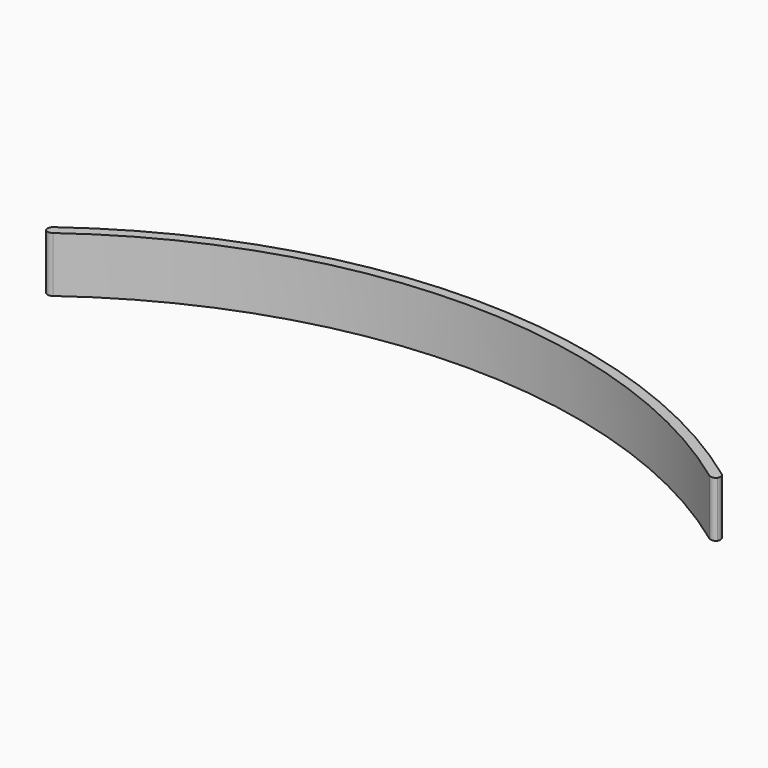
from build123d import *

# Parameters (mm, degrees)
F1_DEPTH    = 25
F2_T1_DEPTH = 37.6241632485
F2_T3_DEPTH = 37.4381172953


# Not quite as in the source:
# - a fillet or chamfer that OpenCascade refuses, or shapes differently, is made with other operations: its cross-section is extruded or revolved along the edge and cut away or added


with BuildPart() as f1:
    # F0 (on Top) → F1 (new body)
    with BuildSketch(Plane.XY):
        with BuildLine():
            ThreePointArc((-150, 0), (0, 50), (150, 0))
            Line((150, 0), (152.7, 3.6))
            ThreePointArc((152.7, 3.6), (0, 54.5), (-152.7, 3.6))
            Line((-152.7, 3.6), (-150, 0))
        make_face()
    extrude(amount=F1_DEPTH)

    # F2: fillet of radius 2.5 on 4 edges, made by hand

    # F2_s2 → F2_t1 (cut)
    with BuildSketch(Plane.XY.offset(-6.3120816242)):
        with BuildLine():
            ThreePointArc((-150.6726442548, 5.1048616519), (-151.6656488685, 3.4559044723), (-151.1925593407, 1.590079121))
            Line((-151.1925593407, 1.590079121), (-152.7, 3.6))
            ThreePointArc((-152.7, 3.6), (-151.6881883097, 4.3549449544), (-150.6726442548, 5.1048616519))
        make_face()
        with BuildLine():
            ThreePointArc((151.1925593407, 1.590079121), (151.6656488685, 3.4559044723), (150.6726442548, 5.1048616519))
            ThreePointArc((150.6726442548, 5.1048616519), (151.6881883097, 4.3549449544), (152.7, 3.6))
            Line((152.7, 3.6), (151.1925593407, 1.590079121))
        make_face()
    extrude(amount=F2_T1_DEPTH, mode=Mode.SUBTRACT)

    # F2_s4 → F2_t3 (cut)
    with BuildSketch(Plane.XY.offset(-6.2190586476)):
        with BuildLine():
            ThreePointArc((-148.0124495796, 1.4753453141), (-149.8583751339, 1.0170056461), (-151.4925740754, 1.9900987672))
            Line((-151.4925740754, 1.9900987672), (-150, 0))
            ThreePointArc((-150, 0), (-149.0080507458, 0.7401325419), (-148.0124495796, 1.4753453141))
        make_face()
        with BuildLine():
            ThreePointArc((148.0124495796, 1.4753453141), (149.8583751339, 1.0170056461), (151.4925740754, 1.9900987672))
            Line((151.4925740754, 1.9900987672), (150, 0))
            ThreePointArc((150, 0), (149.0080507458, 0.7401325419), (148.0124495796, 1.4753453141))
        make_face()
    extrude(amount=F2_T3_DEPTH, mode=Mode.SUBTRACT)


solid = f1.part
